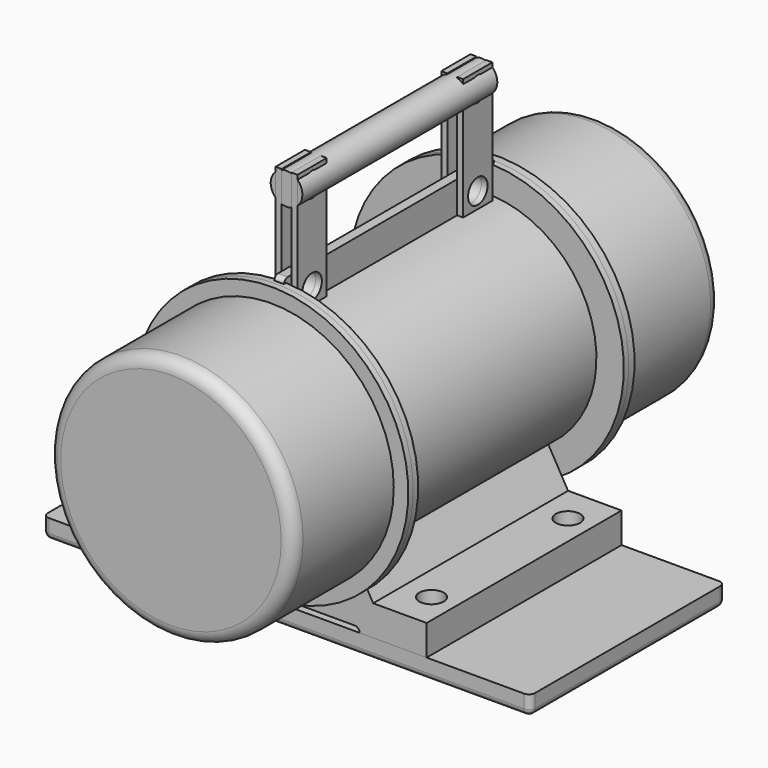
from build123d import *

# Parameters (mm, degrees)
F0_R            = 100.5
F1_DEPTH        = 103
F2_R            = 10
F3_R            = 112.5
F3_R_2          = 100.5
F4_DEPTH        = 5
F5_R            = 112.5
F6_DEPTH        = 5.1
F7_R            = 90
F8_DEPTH        = 211
F9_R            = 112.5
F9_R_2          = 90
F10_DEPTH       = 5
F11_R           = 112.5
F12_DEPTH       = 6
F13_R           = 100.5
F14_DEPTH       = 103
F15_R           = 10
F18_DEPTH       = 100
F19_R           = 10
F20_DEPTH       = 25
F21_W           = 400
F21_H           = 200
F21_R           = 10
F22_DEPTH       = 16
F23_R           = 5
F24_R           = 20
F27_DEPTH       = 2
F28_D           = 20.5
F28_DEPTH       = 25
F28_CSINK_D     = 40
F28_CSINK_ANGLE = 90
F28_TIP         = 6.158821345
F29_R           = 10
F30_DEPTH       = 4
F31_W           = 30
F31_H           = 26.088932828
F31_R           = 10
F31_H_2         = 73.911067172
F32_DEPTH       = 5
F33_W           = 30
F33_H           = 73.911067172
F33_R           = 10
F33_H_2         = 26.088932828
F34_DEPTH       = 5
F35_W           = 200
F35_H           = 13


with BuildPart() as f1:
    # F0 (on Front) → F1 (new body)
    with BuildSketch(Plane.XZ):
        Circle(F0_R)
    extrude(amount=F1_DEPTH)

    # F2
    f2_edges = [f1.edges().sort_by_distance(p)[0] for p in [
        (-100.5, -103, 0),
    ]]
    fillet(f2_edges, radius=F2_R)

    # F3 (on face) → F4 (join)
    with BuildSketch(Plane(origin=(0, 0, 0), x_dir=(-1, 0, 0), z_dir=(0, 1, 0))):
        Circle(F3_R)
        Circle(F3_R_2, mode=Mode.SUBTRACT)
        Circle(F3_R_2)
    extrude(amount=F4_DEPTH)


with BuildPart() as f6:
    # F5 (on face) → F6 (new body)
    with BuildSketch(Plane(origin=(0, 5, 0), x_dir=(-1, 0, 0), z_dir=(0, 1, 0))):
        Circle(F5_R)
    extrude(amount=F6_DEPTH)

    # F7 (on face) → F8 (join)
    with BuildSketch(Plane(origin=(0, 10.1, 0), x_dir=(-1, 0, 0), z_dir=(0, 1, 0))):
        Circle(F7_R)
    extrude(amount=F8_DEPTH)

    # F9 (on face) → F10 (join)
    with BuildSketch(Plane(origin=(0, 221.1, 0), x_dir=(-1, 0, 0), z_dir=(0, 1, 0))):
        Circle(F9_R)
        Circle(F9_R_2, mode=Mode.SUBTRACT)
        Circle(F9_R_2)
    extrude(amount=F10_DEPTH)

    # F17 (on offset) → F18 (join, symmetric)
    with BuildSketch(Plane(origin=(0, 115.6, 0), x_dir=(-1, 0, 0), z_dir=(0, 1, 0))):
        with BuildLine():
            Line((-115, -99.5), (-115, -124.5))
            Line((-115, -124.5), (-60, -124.5))
            ThreePointArc((-60, -124.5), (-58.8284271247, -121.6715728753), (-56, -120.5))
            Line((-56, -120.5), (56, -120.5))
            ThreePointArc((56, -120.5), (58.8284271247, -121.6715728753), (60, -124.5))
            Line((60, -124.5), (115, -124.5))
            Line((115, -124.5), (115, -99.5))
            Line((115, -99.5), (71.1213795416, -99.5))
            Line((71.1213795416, -99.5), (54.8649729171, -71.3430777778))
            ThreePointArc((54.8649729171, -71.3430777778), (0, -90), (-54.8649729171, -71.3430777778))
            Line((-54.8649729171, -71.3430777778), (-71.1213795416, -99.5))
            Line((-71.1213795416, -99.5), (-115, -99.5))
        make_face()
    extrude(amount=F18_DEPTH, both=True)

    # F19 (on face) → F20 (cut)
    with BuildSketch(Plane(origin=(0, 0, -124.5), x_dir=(1, 0, 0), z_dir=(0, 0, -1))):
        with Locations((95, -45.6)):
            Circle(F19_R)
        with Locations((95, -185.6)):
            Circle(F19_R)
        with Locations((-95, -45.6)):
            Circle(F19_R)
        with Locations((-95, -185.6)):
            Circle(F19_R)
    extrude(amount=-F20_DEPTH, mode=Mode.SUBTRACT)

    # F29 (on Right) → F30 (join, symmetric)
    with BuildSketch(Plane.YZ):
        with BuildLine():
            Line((219.807901144, 116), (11.8929979354, 116))
            ThreePointArc((11.8929979354, 116), (9.0645708107, 114.8284271247), (7.8929979354, 112))
            Line((7.8929979354, 112), (7.8929979354, 82))
            Line((7.8929979354, 82), (223.807901144, 82))
            Line((223.807901144, 82), (223.807901144, 112))
            ThreePointArc((223.807901144, 112), (222.6363282688, 114.8284271247), (219.807901144, 116))
        make_face()
        with Locations((30.6, 103)):
            Circle(F29_R, mode=Mode.SUBTRACT)
        with Locations((200.6, 103)):
            Circle(F29_R, mode=Mode.SUBTRACT)
    extrude(amount=F30_DEPTH, both=True)


with BuildPart() as f12:
    # F11 (on face) → F12 (new body)
    with BuildSketch(Plane(origin=(0, 226.1, 0), x_dir=(-1, 0, 0), z_dir=(0, 1, 0))):
        Circle(F11_R)
    extrude(amount=F12_DEPTH)

    # F13 (on face) → F14 (join)
    with BuildSketch(Plane(origin=(0, 232.1, 0), x_dir=(-1, 0, 0), z_dir=(0, 1, 0))):
        Circle(F13_R)
    extrude(amount=F14_DEPTH)

    # F15
    f15_edges = [f12.edges().sort_by_distance(p)[0] for p in [
        (100.5, 335.1, 0),
    ]]
    fillet(f15_edges, radius=F15_R)


with BuildPart() as f22:
    # F21 (on face) → F22 (new body)
    with BuildSketch(Plane(origin=(0, 0, -124.5), x_dir=(1, 0, 0), z_dir=(0, 0, -1))):
        with Locations((0, -115.6)):
            Rectangle(F21_W, F21_H)
        with Locations((-95, -185.6)):
            Circle(F21_R, mode=Mode.SUBTRACT)
        with Locations((95, -185.6)):
            Circle(F21_R, mode=Mode.SUBTRACT)
        with Locations((-95, -45.6)):
            Circle(F21_R, mode=Mode.SUBTRACT)
        with Locations((95, -45.6)):
            Circle(F21_R, mode=Mode.SUBTRACT)
        with Locations((-95, -45.6)):
            Circle(F21_R)
        with Locations((95, -45.6)):
            Circle(F21_R)
        with Locations((95, -185.6)):
            Circle(F21_R)
        with Locations((-95, -185.6)):
            Circle(F21_R)
    extrude(amount=F22_DEPTH)

    # F23
    f23_edges = [f22.edges().sort_by_distance(p)[0] for p in [
        (0, 215.6, -140.5),
        (-200, 115.6, -140.5),
        (0, 15.6, -140.5),
        (200, 115.6, -140.5),
        (-200, 215.6, -132.5),
        (-200, 15.6, -132.5),
        (200, 215.6, -132.5),
        (200, 15.6, -132.5),
    ]]
    fillet(f23_edges, radius=F23_R)

    # F24 (on face) → F27 (cut)
    with BuildSketch(Plane(origin=(0, 0, -140.5), x_dir=(1, 0, 0), z_dir=(0, 0, -1))):
        with Locations((-95, -45.6)):
            Circle(F24_R)
        with Locations((95, -45.6)):
            Circle(F24_R)
        with Locations((-95, -185.6)):
            Circle(F24_R)
        with Locations((95, -185.6)):
            Circle(F24_R)
    extrude(amount=-F27_DEPTH, mode=Mode.SUBTRACT)

    # F28
    with Locations(Plane(origin=(0, 0, -138.5), x_dir=(1, 0, 0), z_dir=(0, 0, -1))):
        with Locations((-95, -45.6), (95, -45.6), (-95, -185.6), (95, -185.6)):
            CounterSinkHole(F28_D / 2, F28_CSINK_D / 2, depth=F28_DEPTH, counter_sink_angle=F28_CSINK_ANGLE)
            with Locations((0, 0, -(F28_DEPTH + F28_TIP / 2))):  # 118° drill point
                Cone(0, F28_D / 2, F28_TIP, mode=Mode.SUBTRACT)


with BuildPart() as f32:
    # F31 (on face) → F32 (new body)
    with BuildSketch(Plane.YZ.offset(4)):
        with Locations((30.6, 102.955533586)):
            Rectangle(F31_W, F31_H)
        with Locations((30.6, 103)):
            Circle(F31_R, mode=Mode.SUBTRACT)
        with Locations((30.6, 152.955533586)):
            Rectangle(F31_W, F31_H_2)
        with Locations((30.6, 176.911067172)):
            Circle(F31_R, mode=Mode.SUBTRACT)
    extrude(amount=F32_DEPTH)


with BuildPart() as f32b:
    # F31 (on face) → F32, piece 2 (new body)
    with BuildSketch(Plane.YZ.offset(4)):
        with Locations((200.6, 102.955533586)):
            Rectangle(F31_W, F31_H)
        with Locations((200.6, 103)):
            Circle(F31_R, mode=Mode.SUBTRACT)
        with Locations((200.6, 152.955533586)):
            Rectangle(F31_W, F31_H_2)
        with Locations((200.6, 176.911067172)):
            Circle(F31_R, mode=Mode.SUBTRACT)
    extrude(amount=F32_DEPTH)


with BuildPart() as f34:
    # F33 (on face) → F34 (new body)
    with BuildSketch(Plane(origin=(-4, 0, 0), x_dir=(0, -1, 0), z_dir=(-1, 0, 0))):
        with Locations((-200.6, 152.955533586)):
            Rectangle(F33_W, F33_H)
        with Locations((-200.6, 176.911067172)):
            Circle(F33_R, mode=Mode.SUBTRACT)
        with Locations((-200.6, 102.955533586)):
            Rectangle(F33_W, F33_H_2)
        with Locations((-200.6, 103)):
            Circle(F33_R, mode=Mode.SUBTRACT)
    extrude(amount=F34_DEPTH)


with BuildPart() as f34b:
    # F33 (on face) → F34, piece 2 (new body)
    with BuildSketch(Plane(origin=(-4, 0, 0), x_dir=(0, -1, 0), z_dir=(-1, 0, 0))):
        with Locations((-30.6, 152.955533586)):
            Rectangle(F33_W, F33_H)
        with Locations((-30.6, 176.911067172)):
            Circle(F33_R, mode=Mode.SUBTRACT)
        with Locations((-30.6, 102.955533586)):
            Rectangle(F33_W, F33_H_2)
        with Locations((-30.6, 103)):
            Circle(F33_R, mode=Mode.SUBTRACT)
    extrude(amount=F34_DEPTH)


with BuildPart() as f36:
    # F35 (on Right) → F36 (revolve)
    with BuildSketch(Plane.YZ):
        with Locations((115.6, 183.411067172)):
            Rectangle(F35_W, F35_H)
    revolve(axis=Axis((0, 115.6, 176.911067172), (0, -1, 0)))

    # F37: cut F34b, F32, F34, F32b
    add(f34b.part, mode=Mode.SUBTRACT)
    add(f32.part, mode=Mode.SUBTRACT)
    add(f34.part, mode=Mode.SUBTRACT)
    add(f32b.part, mode=Mode.SUBTRACT)


solid = Compound([f1.part, f6.part, f12.part, f22.part, f32.part, f32b.part, f34.part, f34b.part, f36.part])
